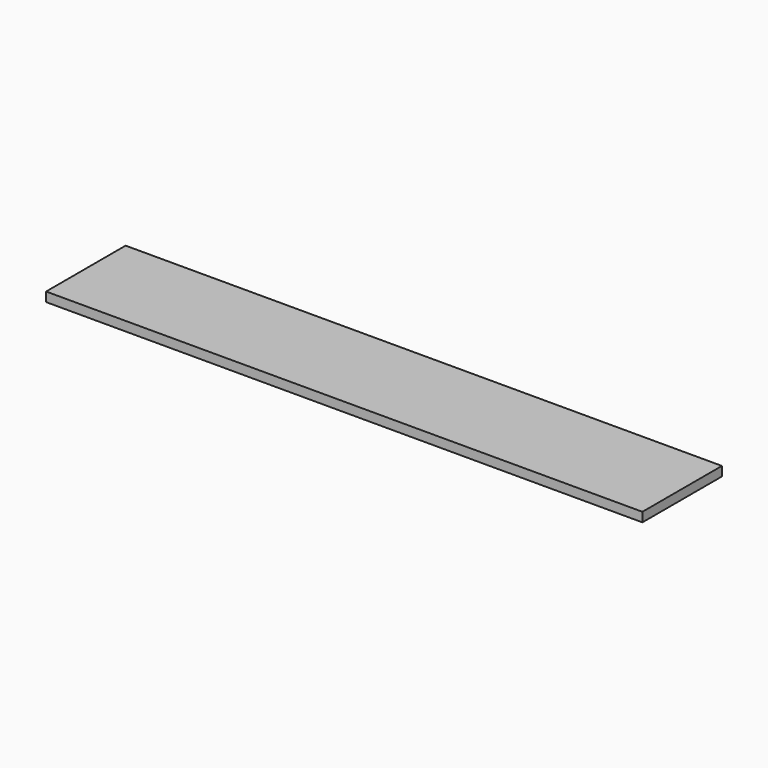
from build123d import *

# Parameters (mm, degrees)
F0_W     = 1219.2
F0_H     = 203.2
F1_DEPTH = 19.05


# Not quite as in the source:
# - a length typed as a fraction of an inch, garbled in the dataset ("3 / 203.2 mm" for 3/8 in), is restored


with BuildPart() as f1:
    # F0 (on Top) → F1 (new body)
    with BuildSketch(Plane.XY):
        Rectangle(F0_W, F0_H)
    extrude(amount=F1_DEPTH)


solid = f1.part
